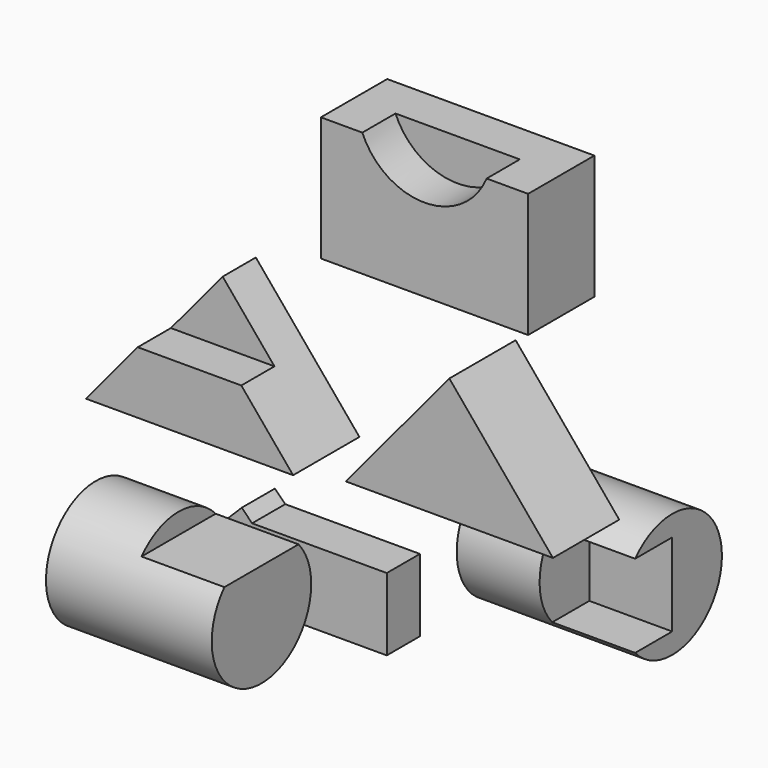
from build123d import *

# Parameters (mm, degrees)
F1_DEPTH  = 25.4
F3_DEPTH  = 12.7
F5_DEPTH  = 25.4
F6_W      = 31.75
F6_H      = 12.7
F7_DEPTH  = 12.7
F8_R      = 19.05
F9_DEPTH  = 50.8
F11_DEPTH = 25.4
F12_R     = 19.05
F13_DEPTH = 50.8
F15_DEPTH = 25.4
F16_W     = 63.5
F16_H     = 38.1000004709
F17_DEPTH = 25.4
F19_DEPTH = 12.7


with BuildPart() as f1:
    # F0 (on Front) → F1 (new body)
    with BuildSketch(Plane.XZ):
        Polygon((-38.1, 38.2058574115), (-69.85, 0.1058574115), (-6.35, 0.1058574115), align=None)
    extrude(amount=F1_DEPTH)

    # F2 (on face) → F3 (cut)
    with BuildSketch(Plane.XZ.offset(25.4)):
        Polygon((-53.975, 19.1558574115), (-38.1, 19.1558574115), (-22.225, 19.1558574115), (-38.1, 38.2058574115), align=None)
    extrude(amount=-F3_DEPTH, mode=Mode.SUBTRACT)


with BuildPart() as f5:
    # F4 (on Front) → F5 (new body)
    with BuildSketch(Plane.XZ):
        Polygon((25.6539984085, 22.7330001045), (9.7789984085, 3.6830001045), (73.2789984085, 3.6830001045), (57.4039984085, 22.7330001045), (41.5289984085, 22.7330001045), align=None)
        Polygon((41.5289984085, 41.7830001045), (25.6539984085, 22.7330001045), (41.5289984085, 22.7330001045), (57.4039984085, 22.7330001045), align=None)
    extrude(amount=F5_DEPTH)


with BuildPart() as f7:
    # F6 (on Front) → F7 (new body)
    with BuildSketch(Plane.XZ):
        Polygon((-39.2430012196, -33.8879922846), (-29.7180012196, -43.4129922846), (2.0319987804, -43.4129922846), (2.0319987804, -33.8879922846), align=None)
        with Locations((-13.8430012196, -49.7629922846)):
            Rectangle(F6_W, F6_H)
        Polygon((-55.1180012196, -43.4129922846), (-55.1180012196, -56.1129922846), (-29.7180012196, -56.1129922846), (-29.7180012196, -43.4129922846), (-39.2430012196, -33.8879922846), (-42.4180012196, -30.7129922846), align=None)
    extrude(amount=-F7_DEPTH)


with BuildPart() as f9:
    # F8 (on Right) → F9 (new body)
    with BuildSketch(Plane.YZ):
        with Locations((-45.4660002142, -26.7969986916)):
            Circle(F8_R)
    extrude(amount=-F9_DEPTH)

    # F10 (on face) → F11 (cut)
    with BuildSketch(Plane.YZ):
        with BuildLine():
            Line((-59.6650318713, -14.0969986916), (-45.4660002142, -14.0969986916))
            Line((-45.4660002142, -14.0969986916), (-31.2669685571, -14.0969986916))
            ThreePointArc((-31.2669685571, -14.0969986916), (-45.4660002142, -7.7469986916), (-59.6650318713, -14.0969986916))
        make_face()
    extrude(amount=-F11_DEPTH, mode=Mode.SUBTRACT)


with BuildPart() as f13:
    # F12 (on Right) → F13 (new body)
    with BuildSketch(Plane.YZ):
        with Locations((48.3870003372, -40.7670012236)):
            Circle(F12_R)
    extrude(amount=F13_DEPTH)

    # F14 (on face) → F15 (cut)
    with BuildSketch(Plane.YZ.offset(50.8)):
        with BuildLine():
            Line((48.3870003372, -53.4670012236), (48.3870003372, -40.7670012236))
            Line((48.3870003372, -40.7670012236), (48.3870003372, -28.0670012236))
            Line((48.3870003372, -28.0670012236), (34.1879686801, -28.0670012236))
            ThreePointArc((34.1879686801, -28.0670012236), (29.3370003372, -40.7670012236), (34.1879686801, -53.4670012236))
            Line((34.1879686801, -53.4670012236), (48.3870003372, -53.4670012236))
        make_face()
    extrude(amount=-F15_DEPTH, mode=Mode.SUBTRACT)


with BuildPart() as f17:
    # F16 (on Front) → F17 (new body)
    with BuildSketch(Plane.XZ):
        with Locations((33.9089920744, 80.3909990937)):
            Rectangle(F16_W, F16_H)
    extrude(amount=F17_DEPTH)

    # F18 (on face) → F19 (cut)
    with BuildSketch(Plane.XZ.offset(25.4)):
        with BuildLine():
            Line((52.9589920744, 99.4409993291), (14.8589920744, 99.4409993291))
            ThreePointArc((14.8589920744, 99.4409993291), (33.9089920744, 86.7409988582), (52.9589920744, 99.4409993291))
        make_face()
    extrude(amount=-F19_DEPTH, mode=Mode.SUBTRACT)


solid = Compound([f1.part, f5.part, f7.part, f9.part, f13.part, f17.part])
